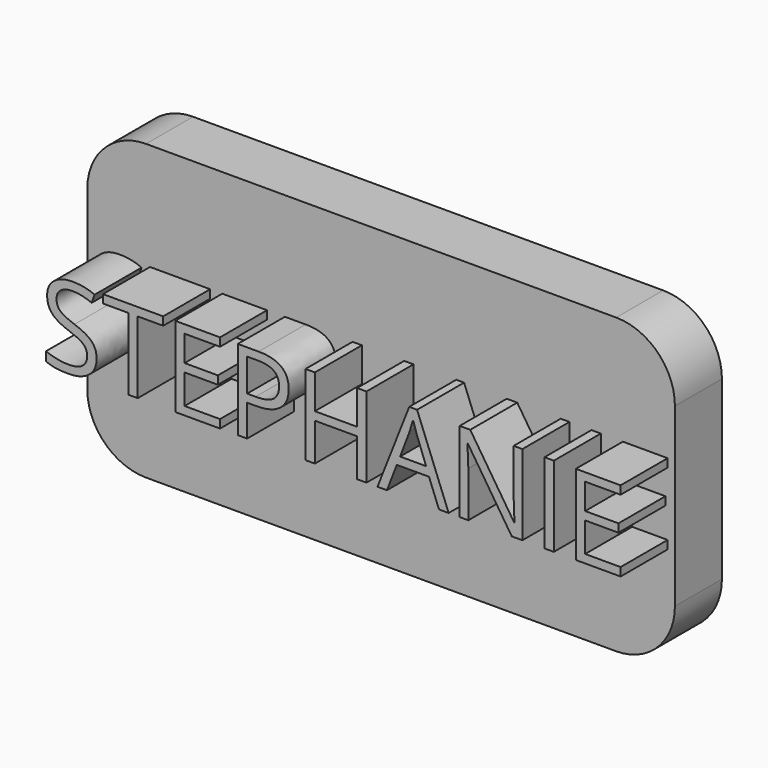
from build123d import *

# Parameters (mm, degrees)
F1_DEPTH     = 10
F2_T         = -1
F3_TEXT_SIZE = 19.1404731286
F4_DEPTH     = 10


# Not quite as in the source:
# - Text() gives the source's letters only with a copy of the font that has no kerning and outlines rounded to 1/6400 em; it was checked with that copy


with BuildPart() as f1:
    # F0 (on Front) → F1 (new body)
    with BuildSketch(Plane.XZ):
        with BuildLine():
            Line((40, 25), (-40, 25))
            ThreePointArc((-40, 25), (-47.0710678119, 22.0710678119), (-50, 15))
            Line((-50, 15), (-50, -15))
            ThreePointArc((-50, -15), (-47.0710678119, -22.0710678119), (-40, -25))
            Line((-40, -25), (40, -25))
            ThreePointArc((40, -25), (47.0710678119, -22.0710678119), (50, -15))
            Line((50, -15), (50, 15))
            ThreePointArc((50, 15), (47.0710678119, 22.0710678119), (40, 25))
        make_face()
    extrude(amount=F1_DEPTH)

    # F2
    f2_openings = [f1.faces().sort_by_distance(p)[0] for p in [
        (0, 0, 0),
    ]]
    offset(amount=F2_T, openings=f2_openings)

    # F3 (on face) → F4 (join)
    with BuildSketch(Plane.XZ.offset(10)):
        with Locations((-50, -6.8905703263)):
            Text('STEPHANIE', F3_TEXT_SIZE, font='Open Sans', text_align=(TextAlign.LEFT, TextAlign.BOTTOM))
    extrude(amount=F4_DEPTH)


solid = f1.part
